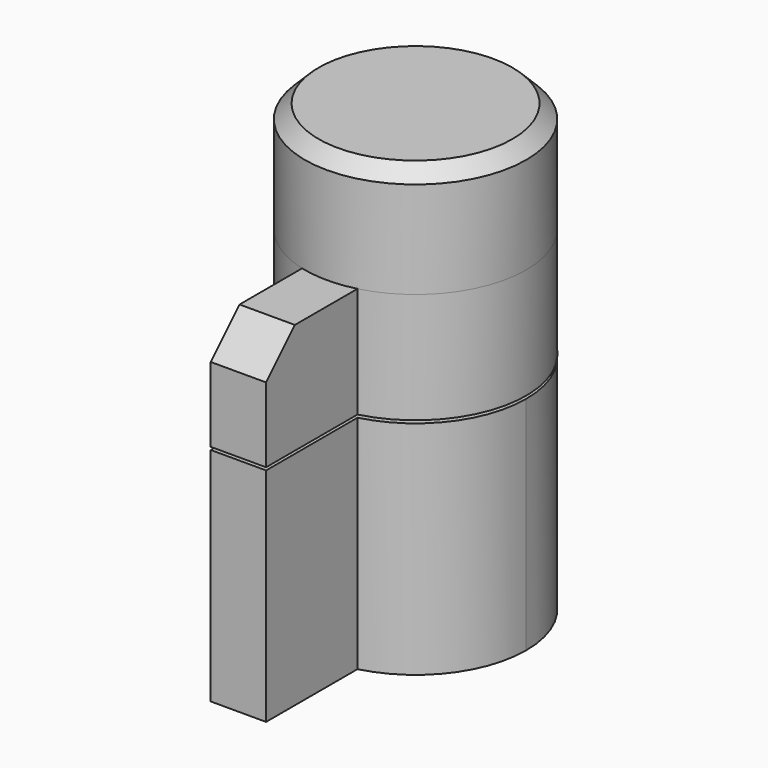
from build123d import *

# Parameters (mm, degrees)
F0_R      = 3
F2_DEPTH  = 8
F3_R      = 2.9
F4_DEPTH  = 8
F5_R      = 2.9
F6_DEPTH  = 0.1
F8_DEPTH  = 4
F9_R      = 4
F10_DEPTH = 4
F11_SIZE  = 1.3
F12_SIZE  = 0.5


with BuildPart() as f2:
    # F0 (on Top) → F2 (new body)
    with BuildSketch(Plane.XY):
        with BuildLine():
            ThreePointArc((1, -3.872983), (3.162278, -2.44949), (4, 0))
            ThreePointArc((4, 0), (-2.44949, 3.162278), (-1, -3.872983))
            ThreePointArc((-1, -3.872983), (0, -4), (1, -3.872983))
        make_face()
        Circle(F0_R, mode=Mode.SUBTRACT)
        with BuildLine():
            ThreePointArc((1, -3.872983), (0, -4), (-1, -3.872983))
            Line((-1, -3.872983), (-1, -8))
            Line((-1, -8), (1, -8))
            Line((1, -8), (1, -3.872983))
        make_face()
    extrude(amount=F2_DEPTH)


with BuildPart() as f4:
    # F3 (on Top) → F4 (new body, through all)
    with BuildSketch(Plane.XY):
        Circle(F3_R)
    extrude(amount=F4_DEPTH)

    # F5 (on face) → F6 (join)
    with BuildSketch(Plane.XY.offset(8)):
        Circle(F5_R)
    extrude(amount=F6_DEPTH)

    # F7 (on face) → F8 (join)
    with BuildSketch(Plane.XY.offset(8.1)):
        with BuildLine():
            Line((1, -8), (1, -3.872983))
            ThreePointArc((1, -3.872983), (0, 4), (-1, -3.872983))
            Line((-1, -3.872983), (-1, -8))
            Line((-1, -8), (1, -8))
        make_face()
    extrude(amount=F8_DEPTH)

    # F9 (on face) → F10 (join)
    with BuildSketch(Plane.XY.offset(12.1)):
        Circle(F9_R)
    extrude(amount=F10_DEPTH)

    # F11
    f11_edges = [f4.edges().sort_by_distance(p)[0] for p in [
        (0, -8, 12.1),
    ]]
    chamfer(f11_edges, length=F11_SIZE)

    # F12
    f12_edges = [f4.edges().sort_by_distance(p)[0] for p in [
        (-4, 0, 16.1),
    ]]
    chamfer(f12_edges, length=F12_SIZE)


solid = Compound([f2.part, f4.part])
